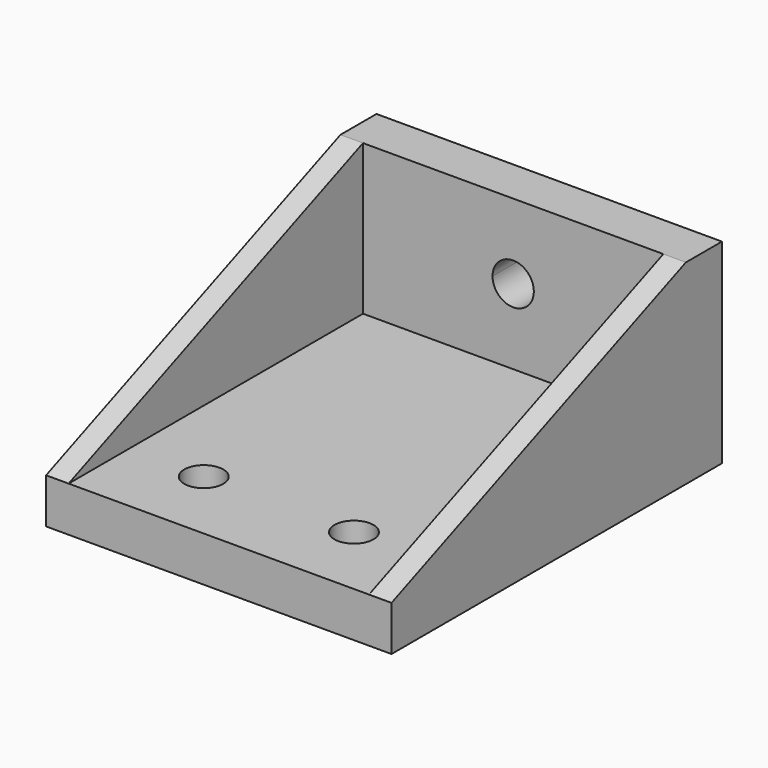
from build123d import *

# Parameters (mm, degrees)
F0_W     = 40
F0_H     = 20
F0_R     = 2.6
F0_H_2   = 29
F1_DEPTH = 6
F0_H_3   = 6
F2_DEPTH = 26
F4_DEPTH = 3
F6_DEPTH = 25


# Not quite as in the source:
# - a pattern or mirror of a feature is missing from the dataset's text; its kind, count and spacing are read off the source's solid


with BuildPart() as f1:
    # F0 (on Top) → F1 (new body)
    with BuildSketch(Plane.XY):
        Rectangle(F0_W, F0_H)
        with Locations((-10, 0)):
            Circle(F0_R, mode=Mode.SUBTRACT)
        with Locations((10, 0)):
            Circle(F0_R, mode=Mode.SUBTRACT)
        with Locations((0, 24.5)):
            Rectangle(F0_W, F0_H_2)
    extrude(amount=F1_DEPTH)

    # F0 (on Top) → F2 (join)
    with BuildSketch(Plane.XY):
        with Locations((0, 42)):
            Rectangle(F0_W, F0_H_3)
    extrude(amount=F2_DEPTH)

    # F3 (on face) → F4 (join)
    with BuildSketch(Plane(origin=(-20, 0, 0), x_dir=(0, -1, 0), z_dir=(-1, 0, 0))):
        Polygon((10, 0), (10, 6), (-39, 26), (-45, 26), (-45, 0), align=None)
    f4 = extrude(amount=F4_DEPTH)

    # F4_copies: F4 across plane
    add(f4.mirror(Plane(origin=(0, 0, 0), x_dir=(0, 0, 1), z_dir=(1, 0, 0))))

    # F5 (on face) → F6 (cut)
    with BuildSketch(Plane(origin=(0, 45, 0), x_dir=(-1, 0, 0), z_dir=(0, 1, 0))):
        with BuildLine():
            ThreePointArc((0, 18.75), (-1.9445436483, 14.0554563517), (2.75, 16))
            ThreePointArc((2.75, 16), (1.9445436483, 17.9445436483), (0, 18.75))
        make_face()
    extrude(amount=-F6_DEPTH, mode=Mode.SUBTRACT)


solid = f1.part
